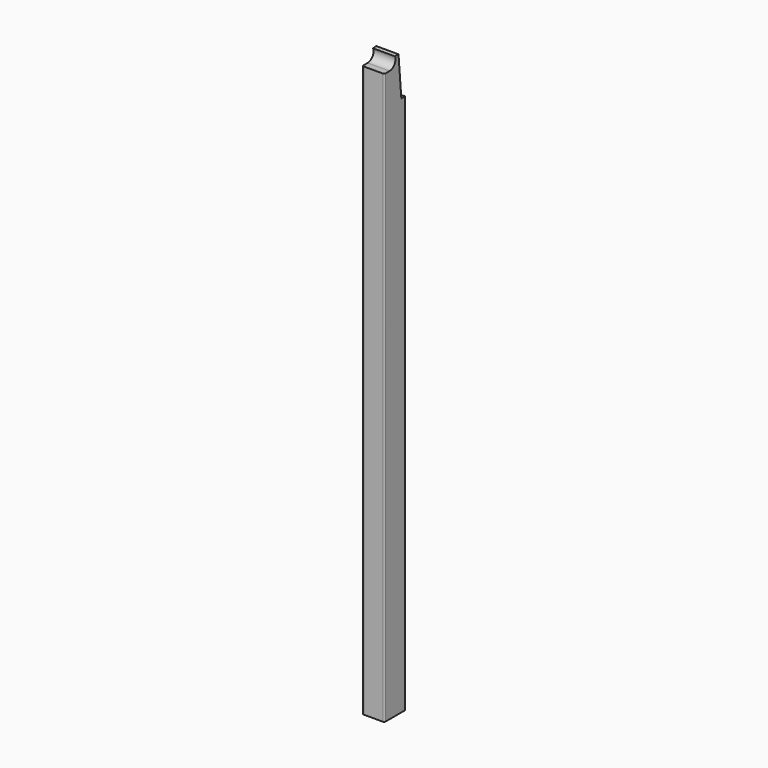
from build123d import *

# Parameters (mm, degrees)
F0_W     = 75
F0_H     = 87.5
F1_DEPTH = 2000
F2_R     = 5
F3_W     = 5
F3_H     = 51
F4_DEPTH = 75.001
F5_R     = 2


# Not quite as in the source:
# - a feature names something its author has since deleted; it is built from what else it names


with BuildPart() as f1:
    # F0 (on Top) → F1 (new body)
    with BuildSketch(Plane.XY):
        Rectangle(F0_W, F0_H)
    extrude(amount=F1_DEPTH)

    # F2
    f2_edges = [f1.edges().sort_by_distance(p)[0] for p in [
        (-37.5, -43.75, 1000),
        (37.5, -43.75, 1000),
    ]]
    fillet(f2_edges, radius=F2_R)

    # F3 (on face) → F4 (cut, through all)
    with BuildSketch(Plane(origin=(-37.5, 0, 0), x_dir=(0, -1, 0), z_dir=(-1, 0, 0))):
        with BuildLine():
            Line((-28.8070795286, 1845.5327422672), (-16.605275544, 1985))
            Line((-16.605275544, 1985), (-1.7898756174, 1983.7038204608))
            ThreePointArc((-1.7898756174, 1983.7038204608), (0.4221879267, 1960.172410035), (21.25, 1949))
            Line((21.25, 1949), (38.75, 1949))
            Line((38.75, 1949), (38.75, 2000))
            Line((38.75, 2000), (-43.75, 2000))
            Line((-43.75, 2000), (-43.75, 1846.8400784084))
            Line((-43.75, 1846.8400784084), (-28.8070795286, 1845.5327422672))
        make_face()
        with Locations((41.25, 1974.5)):
            Rectangle(F3_W, F3_H)
    extrude(amount=-F4_DEPTH, mode=Mode.SUBTRACT)

    # F5
    f5_edges = [f1.edges().sort_by_distance(p)[0] for p in [
        (0, 16.605276, 1985),
        (0, 28.80708, 1845.532742),
    ]]
    fillet(f5_edges, radius=F5_R)


solid = f1.part
